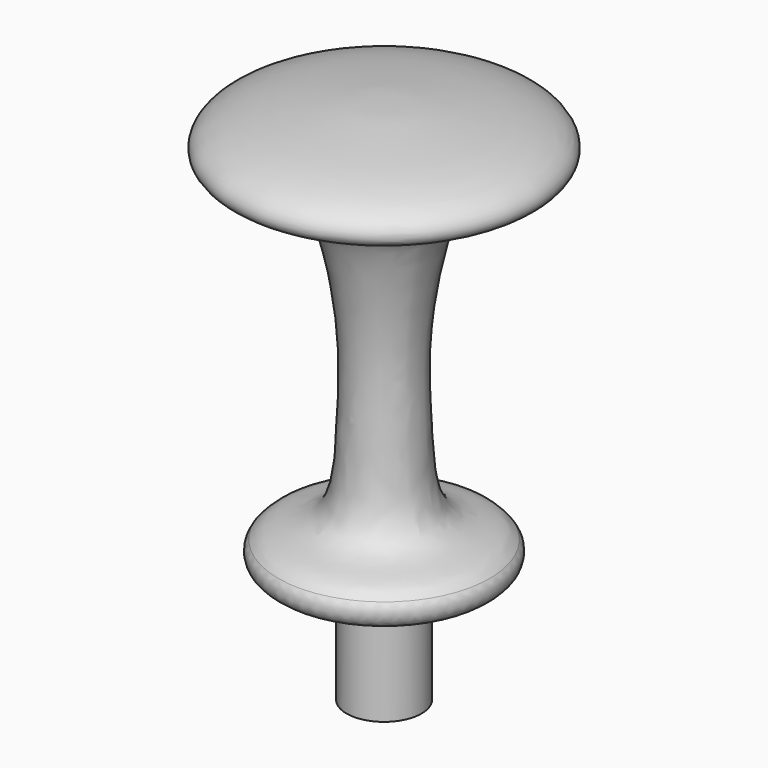
from build123d import *

# Parameters (mm, degrees)
F4_R     = 1.5875
F5_DEPTH = 19.05
F6_R     = 2.54


# Not quite as in the source:
# - a fillet or chamfer that OpenCascade refuses, or shapes differently, is made with other operations: its cross-section is extruded or revolved along the edge and cut away or added


with BuildPart() as f1:
    # F0 (on Front) → F1 (revolve)
    with BuildSketch(Plane.XZ):
        with BuildLine():
            Line((-6.35, 0), (0, 0))
            Line((0, 0), (0, 88.9))
            add(Edge.make_bspline(
                [(-19.05, 22.225), (-17.8315292377, 24.2537166216), (-15.7809404282, 25.8681060581), (-6.9149647749, 26.7821890634), (-6.3387178202, 41.2975869778), (-5.5954996226, 55.3916089231), (-8.721161346, 70.7753261523), (-11.2153222692, 75.0616699951), (-16.8637240899, 78.6093771382), (-26.2709883968, 80.0035727992), (-25.8113743799, 84.1809527212), (-20.748055046, 86.5953556311), (-13.5946930063, 87.8628225206), (-5.5688973368, 88.7420857482), (-3.8394782362, 88.8916157561), (0, 88.9)],
                knots=[0, 0, 0, 0, 0.0626077024, 0.135723906, 0.2346095545, 0.3458708043, 0.4543042288, 0.5143233914, 0.5866708164, 0.6688074457, 0.7134381475, 0.7768461181, 0.8550222886, 0.9294044542, 1, 1, 1, 1], degree=3))
            Line((-19.05, 22.225), (-19.05, 19.05))
            Line((-19.05, 19.05), (-6.35, 19.05))
            Line((-6.35, 19.05), (-6.35, 0))
        make_face()
    revolve(axis=Axis((0, 0, 44.45), (0, 0, 1)))

    # F2: fillet of radius 5.08 on 1 edges, made by hand

    # F2_s1 → F2_t2 (revolve, cut)
    with BuildSketch(Plane.XZ):
        with BuildLine():
            ThreePointArc((-19.05, 22.225), (-17.1805202921, 19.9178865162), (-14.3407139607, 19.05))
            Line((-14.3407139607, 19.05), (-19.05, 19.05))
            Line((-19.05, 19.05), (-19.05, 22.225))
        make_face()
    revolve(axis=Axis((0, 0, 19.05), (0, 0, 1)), mode=Mode.SUBTRACT)

    # F4 (on face) → F5 (cut)
    with BuildSketch(Plane(origin=(0, 0, 0), x_dir=(1, 0, 0), z_dir=(0, 0, -1))):
        Circle(F4_R)
    extrude(amount=-F5_DEPTH, mode=Mode.SUBTRACT)

    # F6
    f6_edges = [f1.edges().sort_by_distance(p)[0] for p in [
        (19.05, 0, 22.225),
    ]]
    fillet(f6_edges, radius=F6_R)


solid = f1.part
